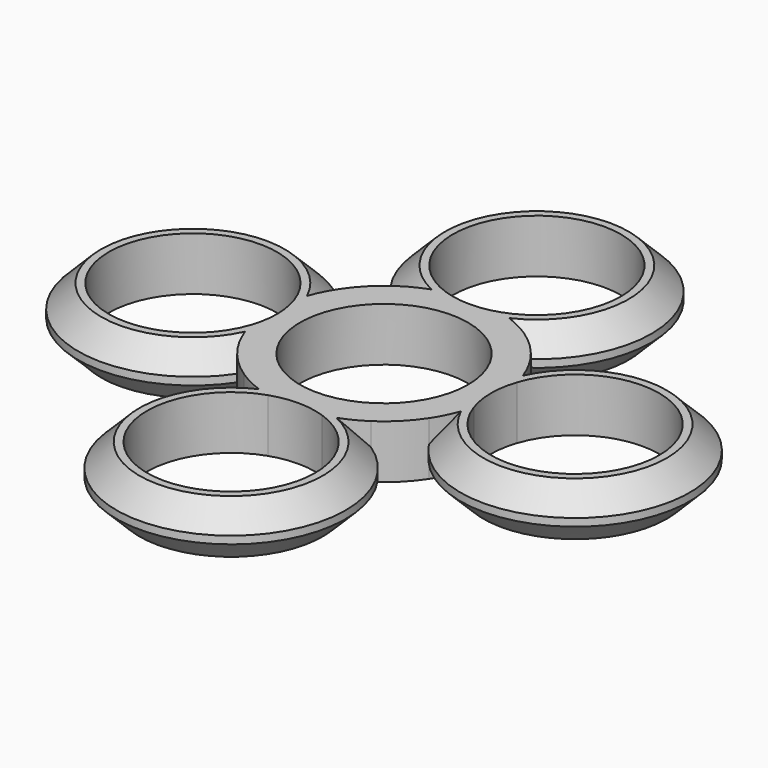
from build123d import *

# Parameters (mm, degrees)
F0_R         = 11.176
F1_DEPTH     = 7.112
F2_T4_ANGLE  = 352.0754293858
F2_S5_R      = 15.24
F2_T6_DEPTH  = 23
F2_T10_ANGLE = 352.0754293858
F2_S11_R     = 15.24
F2_T12_DEPTH = 23
F2_T16_ANGLE = 352.0754293858
F2_S17_R     = 15.24
F2_T18_DEPTH = 23
F2_T22_ANGLE = 352.0754293858
F2_S23_R     = 15.24
F2_T24_DEPTH = 23
F2_T28_ANGLE = 352.0754293858
F2_S29_R     = 15.24
F2_T30_DEPTH = 23
F2_T34_ANGLE = 352.0754293858
F2_S35_R     = 15.24
F2_T36_DEPTH = 23
F2_T40_ANGLE = 352.0754293858
F2_S41_R     = 15.24
F2_T42_DEPTH = 23
F2_T46_ANGLE = 352.0754293858
F2_S47_R     = 15.24
F2_T48_DEPTH = 23


# Not quite as in the source:
# - a fillet or chamfer that OpenCascade refuses, or shapes differently, is made with other operations: its cross-section is extruded or revolved along the edge and cut away or added


with BuildPart() as f1:
    # F0 (on Top) → F1 (new body)
    with BuildSketch(Plane.XY):
        with BuildLine():
            ThreePointArc((-14.224, 0), (-14.3723039868, -1.8146340237), (-14.81328, -3.5811081583))
            ThreePointArc((-14.81328, -3.5811081583), (-13.9681456908, -6.0949574207), (-12.7, -8.4242269675))
            ThreePointArc((-12.7, -8.4242269675), (-10.7763073453, -10.7763073453), (-8.4242269675, -12.7))
            ThreePointArc((-8.4242269675, -12.7), (-6.0949574207, -13.9681456908), (-3.5811081583, -14.81328))
            ThreePointArc((-3.5811081583, -14.81328), (0, -14.224), (3.5811081583, -14.81328))
            ThreePointArc((3.5811081583, -14.81328), (6.0949574207, -13.9681456908), (8.4242269675, -12.7))
            ThreePointArc((8.4242269675, -12.7), (10.7763073453, -10.7763073453), (12.7, -8.4242269675))
            ThreePointArc((12.7, -8.4242269675), (13.9681456908, -6.0949574207), (14.81328, -3.5811081583))
            ThreePointArc((14.81328, -3.5811081583), (14.224, 0), (14.81328, 3.5811081583))
            ThreePointArc((14.81328, 3.5811081583), (13.9681456908, 6.0949574207), (12.7, 8.4242269675))
            ThreePointArc((12.7, 8.4242269675), (10.7763073453, 10.7763073453), (8.4242269675, 12.7))
            ThreePointArc((8.4242269675, 12.7), (6.0949574207, 13.9681456908), (3.5811081583, 14.81328))
            ThreePointArc((3.5811081583, 14.81328), (0, 14.224), (-3.5811081583, 14.81328))
            ThreePointArc((-3.5811081583, 14.81328), (-6.0949574207, 13.9681456908), (-8.4242269675, 12.7))
            ThreePointArc((-8.4242269675, 12.7), (-10.7763073453, 10.7763073453), (-12.7, 8.4242269675))
            ThreePointArc((-12.7, 8.4242269675), (-13.9681456908, 6.0949574207), (-14.81328, 3.5811081583))
            ThreePointArc((-14.81328, 3.5811081583), (-14.3723039868, 1.8146340237), (-14.224, 0))
        make_face()
        Circle(F0_R, mode=Mode.SUBTRACT)
        with BuildLine():
            ThreePointArc((-12.7, -8.4242269675), (-13.9681456908, -6.0949574207), (-14.81328, -3.5811081583))
            ThreePointArc((-14.81328, -3.5811081583), (-36.576, 0), (-14.81328, 3.5811081583))
            ThreePointArc((-14.81328, 3.5811081583), (-13.9681456908, 6.0949574207), (-12.7, 8.4242269675))
            ThreePointArc((-12.7, 8.4242269675), (-40.64, 0), (-12.7, -8.4242269675))
        make_face()
        with BuildLine():
            ThreePointArc((-3.5811081583, -14.81328), (-6.0949574207, -13.9681456908), (-8.4242269675, -12.7))
            ThreePointArc((-8.4242269675, -12.7), (0, -40.64), (8.4242269675, -12.7))
            ThreePointArc((8.4242269675, -12.7), (6.0949574207, -13.9681456908), (3.5811081583, -14.81328))
            ThreePointArc((3.5811081583, -14.81328), (9.0808986553, -18.8853813917), (11.176, -25.4))
            ThreePointArc((11.176, -25.4), (-6.5146186083, -34.4808986553), (-3.5811081583, -14.81328))
        make_face()
        with BuildLine():
            ThreePointArc((8.4242269675, 12.7), (0, 40.64), (-8.4242269675, 12.7))
            ThreePointArc((-8.4242269675, 12.7), (-6.0949574207, 13.9681456908), (-3.5811081583, 14.81328))
            ThreePointArc((-3.5811081583, 14.81328), (-6.5146186083, 34.4808986553), (11.176, 25.4))
            ThreePointArc((11.176, 25.4), (9.0808986553, 18.8853813917), (3.5811081583, 14.81328))
            ThreePointArc((3.5811081583, 14.81328), (6.0949574207, 13.9681456908), (8.4242269675, 12.7))
        make_face()
        with BuildLine():
            ThreePointArc((14.81328, -3.5811081583), (13.9681456908, -6.0949574207), (12.7, -8.4242269675))
            ThreePointArc((12.7, -8.4242269675), (40.64, 0), (12.7, 8.4242269675))
            ThreePointArc((12.7, 8.4242269675), (13.9681456908, 6.0949574207), (14.81328, 3.5811081583))
            ThreePointArc((14.81328, 3.5811081583), (27.2146340237, 11.0276960132), (36.576, 0))
            ThreePointArc((36.576, 0), (27.2146340237, -11.0276960132), (14.81328, -3.5811081583))
        make_face()
    extrude(amount=F1_DEPTH)

    # F2: chamfer of 3.048 on 8 edges, made by hand


with BuildPart() as f2_tool2:
    # F2_s3 → F2_t4 (revolve)
    with BuildSketch(Plane(origin=(1.7509401303, 0.1212795301, 0), x_dir=(0, 0, 1), z_dir=(-0.997609751, -0.0690998166, 0))):
        Polygon((4.064, 10.0992876762), (7.112, 13.1472876762), (7.112, 10.0992876762), align=None)
    revolve(axis=Axis((0, 25.4, 7.112), (0, 0, 1)), revolution_arc=F2_T4_ANGLE)

    # F2_s5 → F2_t6 (cut, symmetric)
    with BuildSketch(Plane.XY.offset(5.6)):
        Circle(F2_S5_R)
    extrude(amount=F2_T6_DEPTH, both=True, mode=Mode.SUBTRACT)


with BuildPart() as f1_1:
    add(f1.part)

    # F2_t1: cut F2_tool2
    add(f2_tool2.part, mode=Mode.SUBTRACT)


with BuildPart() as f2_tool8:
    # F2_s9 → F2_t10 (revolve)
    with BuildSketch(Plane(origin=(1.7509401303, 0.1212795301, 0), x_dir=(0, 0, 1), z_dir=(-0.997609751, -0.0690998166, 0))):
        Polygon((3.048, 10.0992876762), (0, 13.1472876762), (0, 10.0992876762), align=None)
    revolve(axis=Axis((0, 25.4, 0), (0, 0, 1)), revolution_arc=F2_T10_ANGLE)

    # F2_s11 → F2_t12 (cut, symmetric)
    with BuildSketch(Plane.XY.offset(1.5)):
        Circle(F2_S11_R)
    extrude(amount=F2_T12_DEPTH, both=True, mode=Mode.SUBTRACT)


with BuildPart() as f1_2:
    add(f1_1.part)

    # F2_t7: cut F2_tool8
    add(f2_tool8.part, mode=Mode.SUBTRACT)


with BuildPart() as f2_tool14:
    # F2_s15 → F2_t16 (revolve)
    with BuildSketch(Plane(origin=(0.1212795301, -1.7509401303, 0), x_dir=(0, 0, 1), z_dir=(-0.0690998166, 0.997609751, 0))):
        Polygon((4.064, 10.0992876762), (7.112, 13.1472876762), (7.112, 10.0992876762), align=None)
    revolve(axis=Axis((25.4, 0, 7.112), (0, 0, 1)), revolution_arc=F2_T16_ANGLE)

    # F2_s17 → F2_t18 (cut, symmetric)
    with BuildSketch(Plane.XY.offset(5.6)):
        Circle(F2_S17_R)
    extrude(amount=F2_T18_DEPTH, both=True, mode=Mode.SUBTRACT)


with BuildPart() as f1_3:
    add(f1_2.part)

    # F2_t13: cut F2_tool14
    add(f2_tool14.part, mode=Mode.SUBTRACT)


with BuildPart() as f2_tool20:
    # F2_s21 → F2_t22 (revolve)
    with BuildSketch(Plane(origin=(0.1212795301, -1.7509401303, 0), x_dir=(0, 0, 1), z_dir=(-0.0690998166, 0.997609751, 0))):
        Polygon((3.048, 10.0992876762), (0, 13.1472876762), (0, 10.0992876762), align=None)
    revolve(axis=Axis((25.4, 0, 0), (0, 0, 1)), revolution_arc=F2_T22_ANGLE)

    # F2_s23 → F2_t24 (cut, symmetric)
    with BuildSketch(Plane.XY.offset(1.5)):
        Circle(F2_S23_R)
    extrude(amount=F2_T24_DEPTH, both=True, mode=Mode.SUBTRACT)


with BuildPart() as f1_4:
    add(f1_3.part)

    # F2_t19: cut F2_tool20
    add(f2_tool20.part, mode=Mode.SUBTRACT)


with BuildPart() as f2_tool26:
    # F2_s27 → F2_t28 (revolve)
    with BuildSketch(Plane(origin=(-1.7509401303, -0.1212795301, 0), x_dir=(0, 0, 1), z_dir=(0.997609751, 0.0690998166, 0))):
        Polygon((4.064, 10.0992876762), (7.112, 13.1472876762), (7.112, 10.0992876762), align=None)
    revolve(axis=Axis((0, -25.4, 7.112), (0, 0, 1)), revolution_arc=F2_T28_ANGLE)

    # F2_s29 → F2_t30 (cut, symmetric)
    with BuildSketch(Plane.XY.offset(5.6)):
        Circle(F2_S29_R)
    extrude(amount=F2_T30_DEPTH, both=True, mode=Mode.SUBTRACT)


with BuildPart() as f1_5:
    add(f1_4.part)

    # F2_t25: cut F2_tool26
    add(f2_tool26.part, mode=Mode.SUBTRACT)


with BuildPart() as f2_tool32:
    # F2_s33 → F2_t34 (revolve)
    with BuildSketch(Plane(origin=(-1.7509401303, -0.1212795301, 0), x_dir=(0, 0, 1), z_dir=(0.997609751, 0.0690998166, 0))):
        Polygon((3.048, 10.0992876762), (0, 13.1472876762), (0, 10.0992876762), align=None)
    revolve(axis=Axis((0, -25.4, 0), (0, 0, 1)), revolution_arc=F2_T34_ANGLE)

    # F2_s35 → F2_t36 (cut, symmetric)
    with BuildSketch(Plane.XY.offset(1.5)):
        Circle(F2_S35_R)
    extrude(amount=F2_T36_DEPTH, both=True, mode=Mode.SUBTRACT)


with BuildPart() as f1_6:
    add(f1_5.part)

    # F2_t31: cut F2_tool32
    add(f2_tool32.part, mode=Mode.SUBTRACT)


with BuildPart() as f2_tool38:
    # F2_s39 → F2_t40 (revolve)
    with BuildSketch(Plane(origin=(-0.1212795301, 1.7509401303, 0), x_dir=(0, 0, 1), z_dir=(0.0690998166, -0.997609751, 0))):
        Polygon((4.064, 10.0992876762), (7.112, 13.1472876762), (7.112, 10.0992876762), align=None)
    revolve(axis=Axis((-25.4, 0, 7.112), (0, 0, 1)), revolution_arc=F2_T40_ANGLE)

    # F2_s41 → F2_t42 (cut, symmetric)
    with BuildSketch(Plane.XY.offset(5.6)):
        Circle(F2_S41_R)
    extrude(amount=F2_T42_DEPTH, both=True, mode=Mode.SUBTRACT)


with BuildPart() as f1_7:
    add(f1_6.part)

    # F2_t37: cut F2_tool38
    add(f2_tool38.part, mode=Mode.SUBTRACT)


with BuildPart() as f2_tool44:
    # F2_s45 → F2_t46 (revolve)
    with BuildSketch(Plane(origin=(-0.1212795301, 1.7509401303, 0), x_dir=(0, 0, 1), z_dir=(0.0690998166, -0.997609751, 0))):
        Polygon((3.048, 10.0992876762), (0, 13.1472876762), (0, 10.0992876762), align=None)
    revolve(axis=Axis((-25.4, 0, 0), (0, 0, 1)), revolution_arc=F2_T46_ANGLE)

    # F2_s47 → F2_t48 (cut, symmetric)
    with BuildSketch(Plane.XY.offset(1.5)):
        Circle(F2_S47_R)
    extrude(amount=F2_T48_DEPTH, both=True, mode=Mode.SUBTRACT)


with BuildPart() as f1_8:
    add(f1_7.part)

    # F2_t43: cut F2_tool44
    add(f2_tool44.part, mode=Mode.SUBTRACT)


solid = f1_8.part
